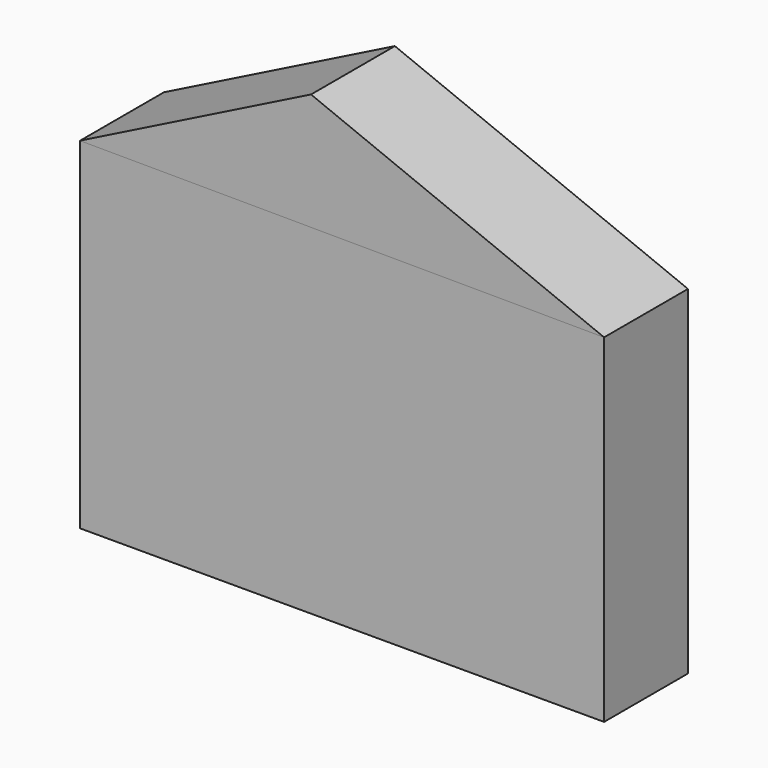
from build123d import *

# Parameters (mm, degrees)
F1_DEPTH = 25.4
F2_W     = 28.4223314375
F2_H     = 15.9875638783
F2_W_2   = 22.6490497589
F2_H_2   = 14.6552654915
F2_W_3   = 21.3167462498
F2_H_3   = 22.2049523145
F2_W_4   = 17.0091595501
F2_H_4   = 31.2147845337
F2_W_5   = 24.8695462942
F2_H_5   = 20.4285569489
F3_DEPTH = 5.08
F5_DEPTH = 25.4


# Not quite as in the source:
# - a feature names something its author has since deleted; it is built from what else it names


with BuildPart() as f1:
    # F0 (on Front) → F1 (new body)
    with BuildSketch(Plane.XZ):
        Polygon((-55.9721749313, 37.4932518983), (-55.9721749313, -45.2112710858), (71.026132632, -45.2112710858), (71.026132632, 36.8376025469), align=None)
    extrude(amount=F1_DEPTH)

    # F2 (on face) → F3 (cut)
    with BuildSketch(Plane(origin=(0, 0, 0), x_dir=(-1, 0, 0), z_dir=(0, 1, 0))):
        with Locations((-37.1482083574, 12.6494523138)):
            Rectangle(F2_W, F2_H)
        with Locations((34.1296754777, 11.0951049719)):
            Rectangle(F2_W_2, F2_H_2)
        with Locations((34.7958272323, -28.2076550648)):
            Rectangle(F2_W_3, F2_H_3)
        with Locations((0.9776009247, -29.6038788189)):
            Rectangle(F2_W_4, F2_H_4)
        with Locations((-38.4805053473, -29.0958527476)):
            Rectangle(F2_W_5, F2_H_5)
    extrude(amount=-F3_DEPTH, mode=Mode.SUBTRACT)


with BuildPart() as f5:
    # F4 (on face) → F5 (new body)
    with BuildSketch(Plane(origin=(0, 0, 0), x_dir=(-1, 0, 0), z_dir=(0, 1, 0))):
        Polygon((0, 65.5519887805), (-71.026132632, 36.8376025469), (55.9721749313, 37.4932518983), align=None)
    extrude(amount=-F5_DEPTH)


solid = Compound([f1.part, f5.part])
